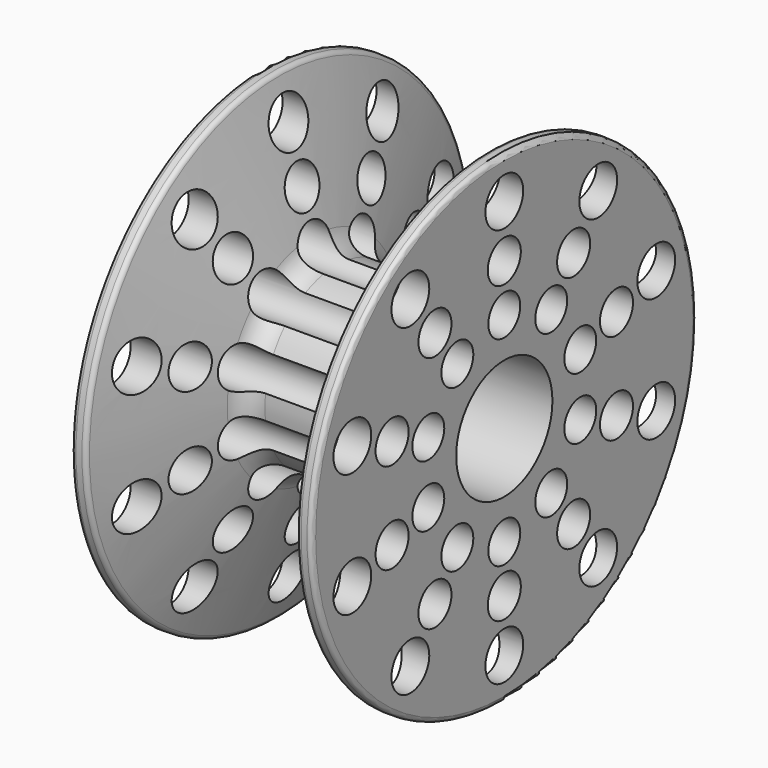
from build123d import *

# Parameters (mm, degrees)
F2_R            = 12.5
F2_R_2          = 5
F3_DEPTH        = 50.001
F4_R            = 4.1465100102
F4_R_2          = 4.2936104376
F4_R_3          = 4.9108149952
F5_DEPTH        = 50.001
F5_COPIES_COUNT = 10


# Not quite as in the source:
# - a pattern or mirror of a feature is missing from the dataset's text; its kind, count and spacing are read off the source's solid


with BuildPart() as f1:
    # F0 (on Top) → F1 (revolve)
    with BuildSketch(Plane.XY):
        with BuildLine():
            Line((25, 5), (25, 49))
            ThreePointArc((25, 49), (24.7071067812, 49.7071067812), (24, 50))
            Line((24, 50), (22.7727354459, 50))
            ThreePointArc((22.7727354459, 50), (22.1612838954, 49.7912818723), (21.8050743906, 49.252254003))
            Line((21.8050743906, 49.252254003), (14.7694562535, 22.2632128315))
            ThreePointArc((14.7694562535, 22.2632128315), (12.9884087291, 19.5680734846), (9.9311509769, 18.5244828463))
            Line((9.9311509769, 18.5244828463), (-9.9311509769, 18.5244828463))
            ThreePointArc((-9.9311509769, 18.5244828463), (-12.9884087291, 19.5680734846), (-14.7694562535, 22.2632128315))
            Line((-14.7694562535, 22.2632128315), (-21.8050743906, 49.252254003))
            ThreePointArc((-21.8050743906, 49.252254003), (-22.1612838954, 49.7912818723), (-22.7727354459, 50))
            Line((-22.7727354459, 50), (-24, 50))
            ThreePointArc((-24, 50), (-24.7071067812, 49.7071067812), (-25, 49))
            Line((-25, 49), (-25, 5))
            Line((-25, 5), (25, 5))
        make_face()
    revolve(axis=Axis((0, 0, 0), (1, 0, 0)))

    # F2 (on face) → F3 (cut, through all)
    with BuildSketch(Plane.YZ.offset(25)):
        Circle(F2_R)
        Circle(F2_R_2, mode=Mode.SUBTRACT)
    extrude(amount=-F3_DEPTH, mode=Mode.SUBTRACT)

    # F4 (on face) → F5 (cut, through all)
    with BuildSketch(Plane.YZ.offset(25)):
        with Locations((0, -20.7543112338)):
            Circle(F4_R)
        with Locations((0, -30.6465532631)):
            Circle(F4_R_2)
        with Locations((0, -41.5086224675)):
            Circle(F4_R_3)
    f5 = extrude(amount=-F5_DEPTH, mode=Mode.SUBTRACT)

    # F5_copies: F5 ×10 about axis
    f5_copies_axis = Axis((0, 0, 0), (1, 0, 0))
    for i in range(1, F5_COPIES_COUNT):
        add(f5.rotate(f5_copies_axis, i * 360 / F5_COPIES_COUNT), mode=Mode.SUBTRACT)


solid = f1.part
